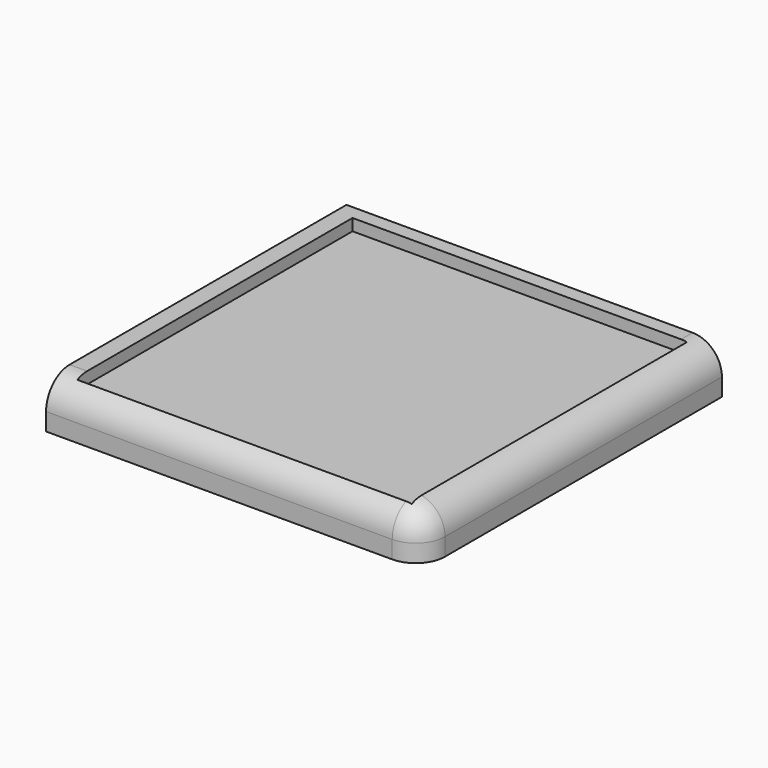
from build123d import *

# Parameters (mm, degrees)
F0_W         = 64
F0_H         = 64
F1_DEPTH     = 6
F2_R         = 3
F3_DEPTH     = 2
F5_DEPTH     = 2
F7_T1_DEPTH  = 71.5
F7_T3_DEPTH  = 15.5
F7_T5_DEPTH  = 71.5
F7_S9_W      = 5
F7_S9_H      = 5
F7_T10_DEPTH = 5


# Not quite as in the source:
# - a fillet or chamfer that OpenCascade refuses, or shapes differently, is made with other operations: its cross-section is extruded or revolved along the edge and cut away or added
# - a feature of the source that left no trace in its solid (it failed there, or was rolled back) is left out


with BuildPart() as f1:
    # F0 (on Top) → F1 (new body)
    with BuildSketch(Plane.XY):
        with Locations((5.897675477, -1.6843453527)):
            Rectangle(F0_W, F0_H)
    extrude(amount=F1_DEPTH)

    # F2 (on Top) → F3 (cut)
    with BuildSketch(Plane.XY):
        with Locations((-16.102324523, 17.3156546473)):
            Circle(F2_R)
        with Locations((-6.1025285926, 17.3795400876)):
            Circle(F2_R)
    extrude(amount=F3_DEPTH, mode=Mode.SUBTRACT)

    # F4 (on face) → F5 (join)
    with BuildSketch(Plane.XY.offset(6)):
        Polygon((-23.111552, 27.8670135885), (-26.102324523, 27.8670135885), (-26.102324523, -33.6843453527), (-23.111552, -33.6843453527), (-23.111552, -30.7656601071), align=None)
        Polygon((-26.102324523, 30.3156546473), (-26.102324523, 27.8670135885), (-23.111552, 27.8670135885), (33.8885635138, 27.8670135885), (37.897675477, 27.8670135885), (37.897675477, 30.3156546473), align=None)
        Polygon((37.897675477, 27.8670135885), (33.8885635138, 27.8670135885), (33.8885635138, -30.7656601071), (37.897675477, -30.7656601071), (37.897675477, -12.6674966887), align=None)
        Polygon((33.8885635138, -30.7656601071), (-23.111552, -30.7656601071), (-23.111552, -33.6843453527), (37.897675477, -33.6843453527), (37.897675477, -30.7656601071), align=None)
    extrude(amount=F5_DEPTH)

    # F7: fillet of radius 5 on 3 edges, made by hand

    # F7_s2 → F7_t1 (cut)
    with BuildSketch(Plane.YZ.offset(-38.602324523)):
        with BuildLine():
            ThreePointArc((-33.6843453527, 3), (-32.2198792586, 6.5355339059), (-28.6843453527, 8))
            Line((-28.6843453527, 8), (-33.6843453527, 8))
            Line((-33.6843453527, 8), (-33.6843453527, 3))
        make_face()
    extrude(amount=F7_T1_DEPTH, mode=Mode.SUBTRACT)

    # F7_s4 → F7_t3 (cut)
    with BuildSketch(Plane.XY.offset(-12.5)):
        with BuildLine():
            ThreePointArc((32.897675477, -33.6843453527), (36.4332093829, -32.2198792586), (37.897675477, -28.6843453527))
            Line((37.897675477, -28.6843453527), (37.897675477, -33.6843453527))
            Line((37.897675477, -33.6843453527), (32.897675477, -33.6843453527))
        make_face()
    extrude(amount=F7_T3_DEPTH, mode=Mode.SUBTRACT)

    # F7_s6 → F7_t5 (cut)
    with BuildSketch(Plane.XZ.offset(-42.8156546473)):
        with BuildLine():
            ThreePointArc((37.897675477, 3), (36.4332093829, 6.5355339059), (32.897675477, 8))
            Line((32.897675477, 8), (37.897675477, 8))
            Line((37.897675477, 8), (37.897675477, 3))
        make_face()
    extrude(amount=F7_T5_DEPTH, mode=Mode.SUBTRACT)


with BuildPart() as f7_tool8:
    # F7_s9 → F7_t10 (new body)
    with BuildSketch(Plane.XZ.offset(28.6843453527)):
        with Locations((35.397675477, 5.5)):
            Rectangle(F7_S9_W, F7_S9_H)
    extrude(amount=F7_T10_DEPTH)

    # F7_s11 → F7_t12 (revolve, cut)
    with BuildSketch(Plane(origin=(32.897675477, -28.6843453527, 3), x_dir=(-0.7071067812, 0, -0.7071067812), z_dir=(-0.7071067812, 0, 0.7071067812))):
        with BuildLine():
            ThreePointArc((0, -5), (5, 0), (0, 5))
            Line((0, 5), (0, -5))
        make_face()
    revolve(axis=Axis((32.897675477, -28.6843453527, 3), (0, -1, 0)), mode=Mode.SUBTRACT)


with BuildPart() as f1_1:
    add(f1.part)

    # F7_t7: cut F7_tool8
    add(f7_tool8.part, mode=Mode.SUBTRACT)


solid = f1_1.part
